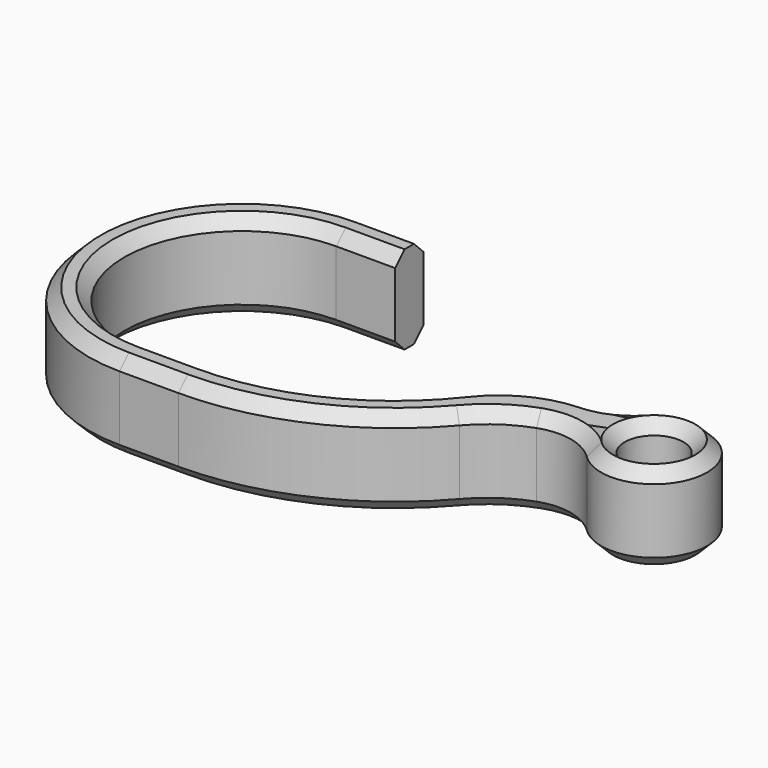
from build123d import *

# Parameters (mm, degrees)
F0_R     = 2.5
F1_DEPTH = 3.75
F2_R     = 5
F3_SIZE  = 0.99999


# Not quite as in the source:
# - a fillet or chamfer is up to 0.001 mm smaller than in the source, because OpenCascade refuses the exact size


with BuildPart() as f1:
    # F0 (on Top) → F1 (new body, symmetric)
    with BuildSketch(Plane.XY):
        with BuildLine():
            ThreePointArc((0, -10), (-10, 0), (0, 10))
            Line((0, 10), (5, 10))
            Line((5, 10), (5, 13))
            Line((5, 13), (0, 13))
            ThreePointArc((0, 13), (-13, 0), (0, -13))
            Line((0, -13), (5, -13))
            ThreePointArc((5, -13), (14.6007417643, -10.9003769721), (22.4486193117, -4.9848484848))
            ThreePointArc((22.4486193117, -4.9848484848), (25.8607399846, -2.4128795773), (30.0349755342, -1.5))
            Line((30.0349755342, -1.5), (30.7573593129, -1.5))
            ThreePointArc((30.7573593129, -1.5), (39.5, 0), (30.7573593129, 1.5))
            Line((30.7573593129, 1.5), (28.6167313572, 1.5))
            ThreePointArc((28.6167313572, 1.5), (24.2387561784, 0.4907359728), (20.7444875715, -2.3333333333))
            ThreePointArc((20.7444875715, -2.3333333333), (13.7559503577, -7.9814719457), (5, -10))
            Line((5, -10), (0, -10))
        make_face()
        with Locations((35, 0)):
            Circle(F0_R, mode=Mode.SUBTRACT)
    extrude(amount=F1_DEPTH, both=True)

    # F2
    f2_edges = [f1.edges().sort_by_distance(p)[0] for p in [
        (30.757359, -1.5, 0),
        (30.757359, 1.5, 0),
    ]]
    fillet(f2_edges, radius=F2_R)

    # F3 (size 1 in the source; OpenCascade refuses exactly that, so slightly less here)
    f3_edges = [f1.edges().sort_by_distance(p)[0] for p in [
        (39.498899, 0.099557, -3.75),
        (39.498899, 0.099557, 3.75),
        (32.5, 0, -3.75),
        (32.5, 0, 3.75),
    ]]
    chamfer(f3_edges, length=F3_SIZE)


solid = f1.part
